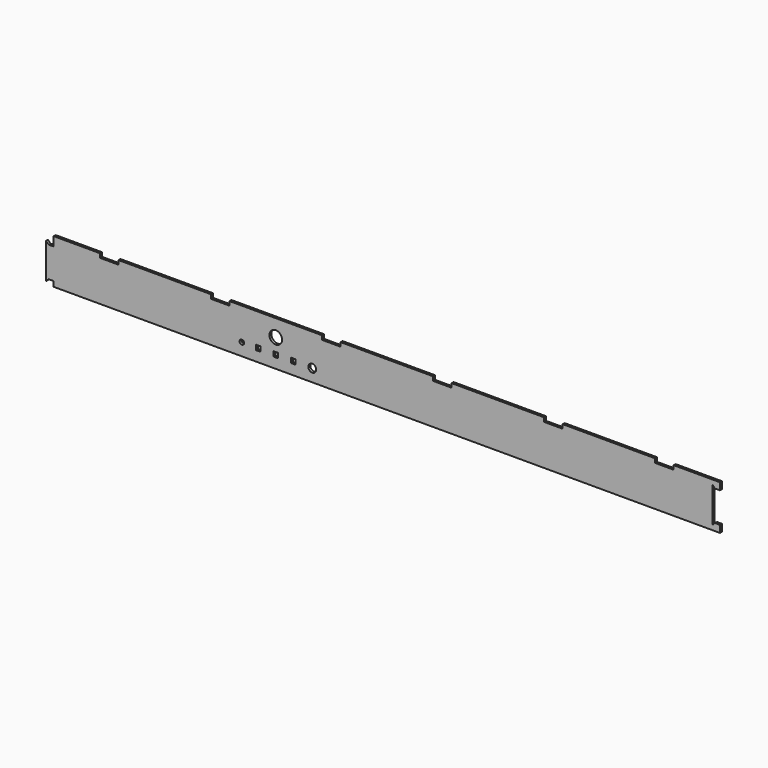
from build123d import *

# Parameters (mm, degrees)
F0_W     = 834.7400754492
F0_H     = 50.8
F1_DEPTH = 3.048
F3_W     = 57.9247
F3_H     = 5.08
F3_W_2   = 115.8494
F4_DEPTH = 3.048
F6_DEPTH = 3.048
F7_DEPTH = 3.049
F8_W     = 6.096
F8_H     = 6.096
F8_R     = 2.8702
F8_R_2   = 4.953
F8_R_3   = 7.9375
F9_DEPTH = 3.049


# Not quite as in the source:
# - a feature names something its author has since deleted; it is built from what else it names


with BuildPart() as f1:
    # F0 (on Front) → F1 (new body)
    with BuildSketch(Plane.XZ):
        with Locations((417.3700377246, 25.4)):
            Rectangle(F0_W, F0_H)
    extrude(amount=F1_DEPTH)

    # F3 (on face) → F4 (join)
    with BuildSketch(Plane.XZ.offset(3.048)):
        with Locations((28.96235, 53.34)):
            Rectangle(F3_W, F3_H)
        with Locations((139.1233459082, 53.34)):
            Rectangle(F3_W_2, F3_H)
        with Locations((278.2466918164, 53.34)):
            Rectangle(F3_W_2, F3_H)
        with Locations((417.3700377246, 53.34)):
            Rectangle(F3_W_2, F3_H)
        with Locations((556.4933836328, 53.34)):
            Rectangle(F3_W_2, F3_H)
        with Locations((695.616729541, 53.34)):
            Rectangle(F3_W_2, F3_H)
        with Locations((805.7777254492, 53.34)):
            Rectangle(F3_W, F3_H)
    extrude(amount=-F4_DEPTH)

    # F5 (on face) → F6 (join)
    with BuildSketch(Plane.XZ.offset(3.048)):
        Polygon((-6.35, 6.35), (0, 6.35), (0, 44.45), (-6.35, 44.45), (-9.525, 47.625), (-9.525, 3.175), align=None)
    extrude(amount=-F6_DEPTH)

    # F5 (on face) → F7 (cut, through all)
    with BuildSketch(Plane.XZ.offset(3.048)):
        Polygon((828.3900754492, 8.89), (834.7400754492, 8.89), (834.7400754492, 46.99), (828.3900754492, 46.99), (825.2150754492, 50.165), (825.2150754492, 5.715), align=None)
    extrude(amount=-F7_DEPTH, mode=Mode.SUBTRACT)

    # F8 (on face) → F9 (cut, through all)
    with BuildSketch(Plane.XZ.offset(3.048)):
        with Locations((256.3264918164, 15.621)):
            Rectangle(F8_W, F8_H)
        with Locations((278.2466918164, 15.621)):
            Rectangle(F8_W, F8_H)
        with Locations((300.1668918164, 15.621)):
            Rectangle(F8_W, F8_H)
        with Locations((235.7016918164, 15.621)):
            Circle(F8_R)
        with Locations((323.9666918164, 15.621)):
            Circle(F8_R_2)
        with Locations((278.2466918164, 34.671)):
            Circle(F8_R_3)
    extrude(amount=-F9_DEPTH, mode=Mode.SUBTRACT)


solid = f1.part
